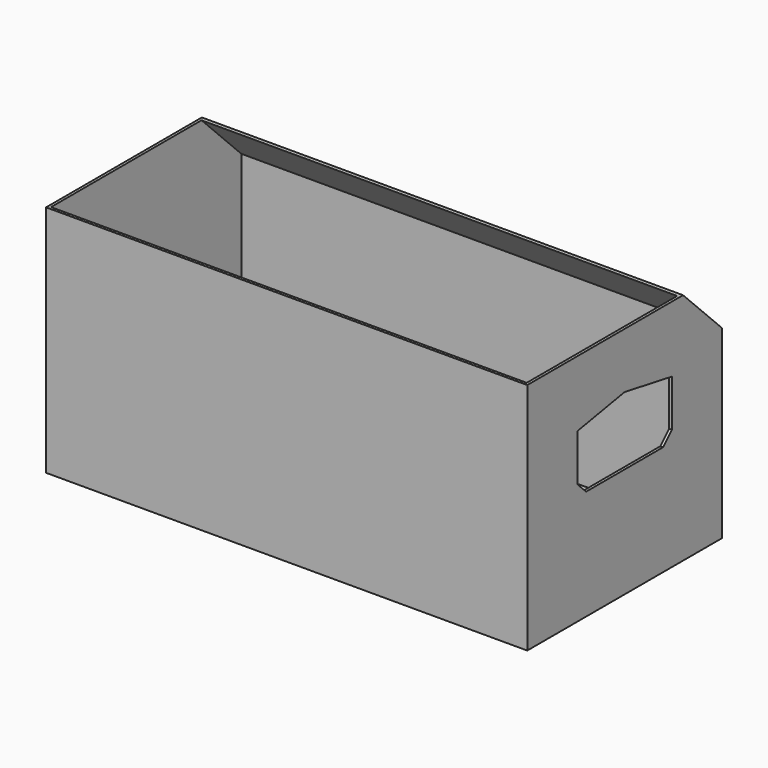
from build123d import *

# Parameters (mm, degrees)
F0_W        = 175
F0_H        = 88.5
F1_DEPTH    = 85
F2_SIZE     = 17.678
F3_T        = -1
F4_W        = 43
F4_H        = 25
F5_DEPTH    = 2
F6_T1_DEPTH = 1
F7_SIZE     = 4


# Not quite as in the source:
# - a fillet or chamfer that OpenCascade refuses, or shapes differently, is made with other operations: its cross-section is extruded or revolved along the edge and cut away or added


with BuildPart() as f1:
    # F0 (on Top) → F1 (new body)
    with BuildSketch(Plane.XY):
        with Locations((87.5, -44.25)):
            Rectangle(F0_W, F0_H)
    extrude(amount=F1_DEPTH)

    # F2
    f2_edges = [f1.edges().sort_by_distance(p)[0] for p in [
        (87.5, 0, 85),
    ]]
    chamfer(f2_edges, length=F2_SIZE)

    # F3
    f3_openings = [f1.faces().sort_by_distance(p)[0] for p in [
        (87.5, -53.089, 85),
    ]]
    offset(amount=F3_T, openings=f3_openings)

    # F4 (on face) → F5 (cut)
    with BuildSketch(Plane.YZ.offset(175)):
        with Locations((-44.25, 52.5)):
            Rectangle(F4_W, F4_H)
    extrude(amount=-F5_DEPTH, mode=Mode.SUBTRACT)

    # F6: chamfer of 4 x 22.6851272785 on 2 edges, made by hand

    # F6_s2 → F6_t1 (join)
    with BuildSketch(Plane.YZ.offset(174)):
        Polygon((-65.75, 61), (-43.0648727215, 65), (-65.75, 65), align=None)
        Polygon((-22.75, 61), (-45.4351272785, 65), (-22.75, 65), align=None)
    extrude(amount=F6_T1_DEPTH)

    # F7
    f7_edges = [f1.edges().sort_by_distance(p)[0] for p in [
        (174.5, -65.75, 40),
        (174.5, -22.75, 40),
    ]]
    chamfer(f7_edges, length=F7_SIZE)


solid = f1.part
